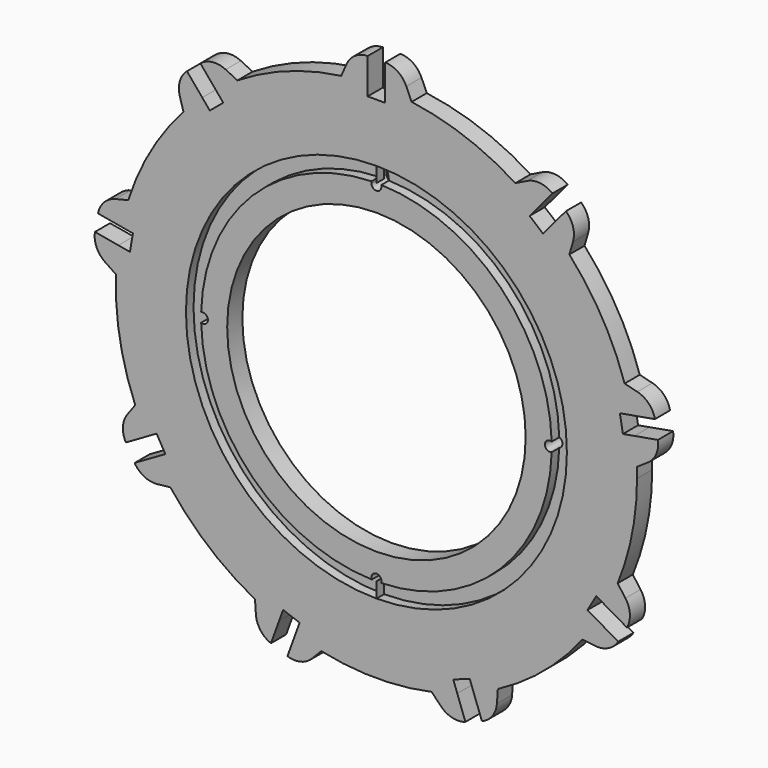
from build123d import *

# Parameters (mm, degrees)
F0_R     = 1.3335
F0_R_2   = 40.005
F1_DEPTH = 5.08
F2_R     = 51.054
F3_DEPTH = 2.54
F5_DEPTH = 2.54


# Not quite as in the source:
# - a pattern or mirror of a feature is missing from the dataset's text; its kind, count and spacing are read off the source's solid


with BuildPart() as f1:
    # F0 (on Front) → F1 (new body)
    with BuildSketch(Plane.XZ):
        with BuildLine():
            ThreePointArc((64.6559292996, -26.4316724103), (68.5391828138, -13.4685900974), (69.85, 0))
            ThreePointArc((69.85, 0), (69.8367147463, 1.3622677557), (69.796864039, 2.7240173131))
            ThreePointArc((69.796864039, 2.7240173131), (69.5676178372, 6.2744759504), (69.1578829213, 9.8086558631))
            Line((69.1578829213, 9.8086558631), (66.0700433255, 9.2641864302))
            Line((66.0700433255, 9.2641864302), (65.2540705387, 13.8917980616))
            Line((65.2540705387, 13.8917980616), (68.3419101345, 14.4362674945))
            ThreePointArc((68.3419101345, 14.4362674945), (67.5181742912, 17.8974478736), (66.5192668833, 21.3121944743))
            ThreePointArc((66.5192668833, 21.3121944743), (60.4918744543, 34.925), (51.7165352668, 46.9512777249))
            ThreePointArc((51.7165352668, 46.9512777249), (49.258731667, 49.5237302165), (46.6731294533, 51.9676965724))
            Line((46.6731294533, 51.9676965724), (44.657685295, 49.565783756))
            Line((44.657685295, 49.565783756), (41.0580424567, 52.5862427339))
            Line((41.0580424567, 52.5862427339), (43.0734866151, 54.9881555503))
            ThreePointArc((43.0734866151, 54.9881555503), (40.2176644871, 57.1100863526), (37.257500213, 59.0838487057))
            ThreePointArc((37.257500213, 59.0838487057), (23.8901070113, 65.6375295619), (9.4374648779, 69.2095134839))
            ThreePointArc((9.4374648779, 69.2095134839), (5.9011375, 69.6002807193), (2.3495, 69.8104744988))
            Line((2.3495, 69.8104744988), (2.3495, 66.675))
            Line((2.3495, 66.675), (-2.3495, 66.675))
            Line((-2.3495, 66.675), (-2.3495, 69.8104744988))
            ThreePointArc((-2.3495, 69.8104744988), (-5.9011375, 69.6002807193), (-9.4374648779, 69.2095134839))
            ThreePointArc((-9.4374648779, 69.2095134839), (-23.8901070113, 65.6375295619), (-37.257500213, 59.0838487057))
            ThreePointArc((-37.257500213, 59.0838487057), (-40.2176644871, 57.1100863526), (-43.0734866151, 54.9881555503))
            Line((-43.0734866151, 54.9881555503), (-41.0580424567, 52.5862427339))
            Line((-41.0580424567, 52.5862427339), (-44.657685295, 49.565783756))
            Line((-44.657685295, 49.565783756), (-46.6731294533, 51.9676965724))
            ThreePointArc((-46.6731294533, 51.9676965724), (-49.258731667, 49.5237302165), (-51.7165352668, 46.9512777249))
            ThreePointArc((-51.7165352668, 46.9512777249), (-60.4918744543, 34.925), (-66.5192668833, 21.3121944743))
            ThreePointArc((-66.5192668833, 21.3121944743), (-67.5181742912, 17.8974478736), (-68.3419101345, 14.4362674945))
            Line((-68.3419101345, 14.4362674945), (-65.2540705387, 13.8917980616))
            Line((-65.2540705387, 13.8917980616), (-66.0700433255, 9.2641864302))
            Line((-66.0700433255, 9.2641864302), (-69.1578829213, 9.8086558631))
            ThreePointArc((-69.1578829213, 9.8086558631), (-69.5676178372, 6.2744759504), (-69.796864039, 2.7240173131))
            ThreePointArc((-69.796864039, 2.7240173131), (-68.7888215479, -12.12932521), (-64.6559292996, -26.4316724103))
            ThreePointArc((-64.6559292996, -26.4316724103), (-63.2261799634, -29.6896053734), (-61.6323943662, -32.8705105632))
            Line((-61.6323943662, -32.8705105632), (-58.9169937973, -31.3027733138))
            Line((-58.9169937973, -31.3027733138), (-56.5674937973, -35.3722266862))
            Line((-56.5674937973, -35.3722266862), (-59.2828943662, -36.9399639356))
            ThreePointArc((-59.2828943662, -36.9399639356), (-57.3250424634, -39.9106753459), (-55.2184644216, -42.7778410736))
            ThreePointArc((-55.2184644216, -42.7778410736), (-44.8987145366, -53.5082043519), (-32.539363826, -61.8078660188))
            ThreePointArc((-32.539363826, -61.8078660188), (-29.3499533501, -63.384562303), (-26.0843963063, -64.7968114134))
            Line((-26.0843963063, -64.7968114134), (-25.0120008688, -61.8504291642))
            Line((-25.0120008688, -61.8504291642), (-20.5963852437, -63.4575818176))
            Line((-20.5963852437, -63.4575818176), (-21.6687806812, -66.4039640668))
            ThreePointArc((-21.6687806812, -66.4039640668), (-18.2594426241, -67.4211780901), (-14.8027316165, -68.2634721992))
            ThreePointArc((-14.8027316165, -68.2634721992), (0, -69.85), (14.8027316165, -68.2634721992))
            ThreePointArc((14.8027316165, -68.2634721992), (18.2594426241, -67.4211780901), (21.6687806812, -66.4039640668))
            Line((21.6687806812, -66.4039640668), (20.5963852437, -63.4575818176))
            Line((20.5963852437, -63.4575818176), (25.0120008688, -61.8504291642))
            Line((25.0120008688, -61.8504291642), (26.0843963063, -64.7968114134))
            ThreePointArc((26.0843963063, -64.7968114134), (29.3499533501, -63.384562303), (32.539363826, -61.8078660188))
            ThreePointArc((32.539363826, -61.8078660188), (44.8987145366, -53.5082043519), (55.2184644216, -42.7778410736))
            ThreePointArc((55.2184644216, -42.7778410736), (57.3250424634, -39.9106753459), (59.2828943662, -36.9399639356))
            Line((59.2828943662, -36.9399639356), (56.5674937973, -35.3722266862))
            Line((56.5674937973, -35.3722266862), (58.9169937973, -31.3027733138))
            Line((58.9169937973, -31.3027733138), (61.6323943662, -32.8705105632))
            ThreePointArc((61.6323943662, -32.8705105632), (63.2261799634, -29.6896053734), (64.6559292996, -26.4316724103))
        make_face()
        with Locations((-46.4947, 0)):
            Circle(F0_R, mode=Mode.SUBTRACT)
        with Locations((0, -46.4947)):
            Circle(F0_R, mode=Mode.SUBTRACT)
        Circle(F0_R_2, mode=Mode.SUBTRACT)
        with Locations((46.4947, 0)):
            Circle(F0_R, mode=Mode.SUBTRACT)
        with BuildLine():
            ThreePointArc((1.3333628788, 46.4755771511), (0, 45.1612), (-1.3333628788, 46.4755771511))
            ThreePointArc((-1.3333628788, 46.4755771511), (-1.0083284803, 48.7431296807), (0, 50.8))
            ThreePointArc((0, 50.8), (1.0083284803, 48.7431296807), (1.3333628788, 46.4755771511))
        make_face(mode=Mode.SUBTRACT)
        with BuildLine():
            ThreePointArc((-43.0734866151, 54.9881555503), (-40.2176644871, 57.1100863526), (-37.257500213, 59.0838487057))
            Line((-37.257500213, 59.0838487057), (-40.4029688253, 60.6296034594))
            ThreePointArc((-40.4029688253, 60.6296034594), (-43.9001960603, 61.242248794), (-47.1796486938, 59.8816889594))
            Line((-47.1796486938, 59.8816889594), (-43.0734866151, 54.9881555503))
        make_face()
        with BuildLine():
            ThreePointArc((-51.7165352668, 46.9512777249), (-49.258731667, 49.5237302165), (-46.6731294533, 51.9676965724))
            Line((-46.6731294533, 51.9676965724), (-50.779291532, 56.8612299815))
            ThreePointArc((-50.779291532, 56.8612299815), (-52.6886523792, 53.8678583382), (-52.69260164, 50.3173770972))
            Line((-52.69260164, 50.3173770972), (-51.7165352668, 46.9512777249))
        make_face()
        with BuildLine():
            ThreePointArc((-9.4374648779, 69.2095134839), (-5.9011375, 69.6002807193), (-2.3495, 69.8104744988))
            Line((-2.3495, 69.8104744988), (-2.3495, 76.1985286816))
            ThreePointArc((-2.3495, 76.1985286816), (-5.7362574703, 75.1327864631), (-8.0214881298, 72.415498574))
            Line((-8.0214881298, 72.415498574), (-9.4374648779, 69.2095134839))
        make_face()
        with BuildLine():
            ThreePointArc((2.3495, 69.8104744988), (5.9011375, 69.6002807193), (9.4374648779, 69.2095134839))
            Line((9.4374648779, 69.2095134839), (8.0214881298, 72.415498574))
            ThreePointArc((8.0214881298, 72.415498574), (5.7362574703, 75.1327864631), (2.3495, 76.1985286816))
            Line((2.3495, 76.1985286816), (2.3495, 69.8104744988))
        make_face()
        with BuildLine():
            ThreePointArc((37.257500213, 59.0838487057), (40.2176644871, 57.1100863526), (43.0734866151, 54.9881555503))
            Line((43.0734866151, 54.9881555503), (47.1796486938, 59.8816889594))
            ThreePointArc((47.1796486938, 59.8816889594), (43.9001960603, 61.242248794), (40.4029688253, 60.6296034594))
            Line((40.4029688253, 60.6296034594), (37.257500213, 59.0838487057))
        make_face()
        with BuildLine():
            ThreePointArc((46.6731294533, 51.9676965724), (49.258731667, 49.5237302165), (51.7165352668, 46.9512777249))
            Line((51.7165352668, 46.9512777249), (52.69260164, 50.3173770972))
            ThreePointArc((52.69260164, 50.3173770972), (52.6886523792, 53.8678583382), (50.779291532, 56.8612299815))
            Line((50.779291532, 56.8612299815), (46.6731294533, 51.9676965724))
        make_face()
        with BuildLine():
            ThreePointArc((66.5192668833, 21.3121944743), (67.5181742912, 17.8974478736), (68.3419101345, 14.4362674945))
            Line((68.3419101345, 14.4362674945), (74.6329154204, 15.5455414622))
            ThreePointArc((74.6329154204, 15.5455414622), (72.9952599579, 18.6957822824), (69.922427638, 20.4744430631))
            Line((69.922427638, 20.4744430631), (66.5192668833, 21.3121944743))
        make_face()
        with BuildLine():
            ThreePointArc((69.1578829213, 9.8086558631), (69.5676178372, 6.2744759504), (69.796864039, 2.7240173131))
            Line((69.796864039, 2.7240173131), (72.7082612299, 4.6751956613))
            ThreePointArc((72.7082612299, 4.6751956613), (74.9874412706, 7.3975606223), (75.4488882072, 10.9179298308))
            Line((75.4488882072, 10.9179298308), (69.1578829213, 9.8086558631))
        make_face()
        with BuildLine():
            Line((66.7244054577, -29.2609367904), (64.6559292996, -26.4316724103))
            ThreePointArc((64.6559292996, -26.4316724103), (63.2261799634, -29.6896053734), (61.6323943662, -32.8705105632))
            Line((61.6323943662, -32.8705105632), (67.1646115693, -36.0645376546))
            ThreePointArc((67.1646115693, -36.0645376546), (67.9350304693, -32.5986485396), (66.7244054577, -29.2609367904))
        make_face()
        with BuildLine():
            Line((64.8151115693, -40.133991027), (59.2828943662, -36.9399639356))
            ThreePointArc((59.2828943662, -36.9399639356), (57.3250424634, -39.9106753459), (55.2184644216, -42.7778410736))
            Line((55.2184644216, -42.7778410736), (58.7029173279, -43.1545617836))
            ThreePointArc((58.7029173279, -43.1545617836), (62.198772999, -42.5341379235), (64.8151115693, -40.133991027))
        make_face()
        with BuildLine():
            Line((23.8536238884, -72.4067714436), (21.6687806812, -66.4039640668))
            ThreePointArc((21.6687806812, -66.4039640668), (18.2594426241, -67.4211780901), (14.8027316165, -68.2634721992))
            Line((14.8027316165, -68.2634721992), (17.229825998, -70.7918201604))
            ThreePointArc((17.229825998, -70.7918201604), (20.3066075788, -72.5636406206), (23.8536238884, -72.4067714436))
        make_face()
        with BuildLine():
            Line((32.3052924046, -65.3047991207), (32.539363826, -61.8078660188))
            ThreePointArc((32.539363826, -61.8078660188), (29.3499533501, -63.384562303), (26.0843963063, -64.7968114134))
            Line((26.0843963063, -64.7968114134), (28.2692395134, -70.7996187901))
            ThreePointArc((28.2692395134, -70.7996187901), (31.0872452104, -68.6398094163), (32.3052924046, -65.3047991207))
        make_face()
        with BuildLine():
            Line((-28.2692395134, -70.7996187901), (-26.0843963063, -64.7968114134))
            ThreePointArc((-26.0843963063, -64.7968114134), (-29.3499533501, -63.384562303), (-32.539363826, -61.8078660188))
            Line((-32.539363826, -61.8078660188), (-32.3052924046, -65.3047991207))
            ThreePointArc((-32.3052924046, -65.3047991207), (-31.0872452104, -68.6398094163), (-28.2692395134, -70.7996187901))
        make_face()
        with BuildLine():
            Line((-17.229825998, -70.7918201604), (-14.8027316165, -68.2634721992))
            ThreePointArc((-14.8027316165, -68.2634721992), (-18.2594426241, -67.4211780901), (-21.6687806812, -66.4039640668))
            Line((-21.6687806812, -66.4039640668), (-23.8536238884, -72.4067714436))
            ThreePointArc((-23.8536238884, -72.4067714436), (-20.3066075788, -72.5636406206), (-17.229825998, -70.7918201604))
        make_face()
        with BuildLine():
            Line((-58.7029173279, -43.1545617836), (-55.2184644216, -42.7778410736))
            ThreePointArc((-55.2184644216, -42.7778410736), (-57.3250424634, -39.9106753459), (-59.2828943662, -36.9399639356))
            Line((-59.2828943662, -36.9399639356), (-64.8151115693, -40.133991027))
            ThreePointArc((-64.8151115693, -40.133991027), (-62.198772999, -42.5341379235), (-58.7029173279, -43.1545617836))
        make_face()
        with BuildLine():
            Line((-67.1646115693, -36.0645376546), (-61.6323943662, -32.8705105632))
            ThreePointArc((-61.6323943662, -32.8705105632), (-63.2261799634, -29.6896053734), (-64.6559292996, -26.4316724103))
            Line((-64.6559292996, -26.4316724103), (-66.7244054577, -29.2609367904))
            ThreePointArc((-66.7244054577, -29.2609367904), (-67.9350304693, -32.5986485396), (-67.1646115693, -36.0645376546))
        make_face()
        with BuildLine():
            Line((-72.7082612299, 4.6751956613), (-69.796864039, 2.7240173131))
            ThreePointArc((-69.796864039, 2.7240173131), (-69.5676178372, 6.2744759504), (-69.1578829213, 9.8086558631))
            Line((-69.1578829213, 9.8086558631), (-75.4488882072, 10.9179298308))
            ThreePointArc((-75.4488882072, 10.9179298308), (-74.9874412706, 7.3975606223), (-72.7082612299, 4.6751956613))
        make_face()
        with BuildLine():
            ThreePointArc((-68.3419101345, 14.4362674945), (-67.5181742912, 17.8974478736), (-66.5192668833, 21.3121944743))
            Line((-66.5192668833, 21.3121944743), (-69.922427638, 20.4744430631))
            ThreePointArc((-69.922427638, 20.4744430631), (-72.9952599579, 18.6957822824), (-74.6329154204, 15.5455414622))
            Line((-74.6329154204, 15.5455414622), (-68.3419101345, 14.4362674945))
        make_face()
    extrude(amount=F1_DEPTH)

    # F2 (on face) → F3 (cut)
    with BuildSketch(Plane.XZ.offset(5.08)):
        Circle(F2_R)
        with BuildLine():
            ThreePointArc((1.3237188184, 46.9713515719), (33.2549291255, 33.1989425865), (46.9735153237, 1.2445714667))
            ThreePointArc((46.9735153237, 1.2445714667), (47.5939548576, 0.7548913882), (47.8282, 0))
            ThreePointArc((47.8282, 0), (47.5939548576, -0.7548913882), (46.9735153237, -1.2445714667))
            ThreePointArc((46.9735153237, -1.2445714667), (33.226947648, -33.226947648), (1.2445714667, -46.9735153237))
            ThreePointArc((1.2445714667, -46.9735153237), (0, -47.8282), (-1.2445714667, -46.9735153237))
            ThreePointArc((-1.2445714667, -46.9735153237), (-33.226947648, -33.226947648), (-46.9735153237, -1.2445714667))
            ThreePointArc((-46.9735153237, -1.2445714667), (-47.8282, 0), (-46.9735153237, 1.2445714667))
            ThreePointArc((-46.9735153237, 1.2445714667), (-33.2549291255, 33.1989425865), (-1.3237188184, 46.9713515719))
            ThreePointArc((-1.3237188184, 46.9713515719), (-0.9312725034, 48.9788228036), (0, 50.8))
            ThreePointArc((0, 50.8), (0.9312725034, 48.9788228036), (1.3237188184, 46.9713515719))
        make_face(mode=Mode.SUBTRACT)
    extrude(amount=-F3_DEPTH, mode=Mode.SUBTRACT)

    # F4 (on face) → F5 (join, through all)
    with BuildSketch(Plane.XZ.offset(5.08)):
        with BuildLine():
            ThreePointArc((0.0254, 51.0539936816), (0, 51.054), (-0.0254, 51.0539936816))
            Line((-0.0254, 51.0539936816), (-0.0254, 46.9899931351))
            ThreePointArc((-0.0254, 46.9899931351), (0, 46.99), (0.0254, 46.9899931351))
            Line((0.0254, 46.9899931351), (0.0254, 51.0539936816))
        make_face()
    f5 = extrude(amount=-F5_DEPTH)

    # F5_copies: F5 across plane
    add(f5.mirror(Plane(origin=(0, 0, 0), x_dir=(-1, 0, 0), z_dir=(0, 0, -1))))


solid = f1.part
